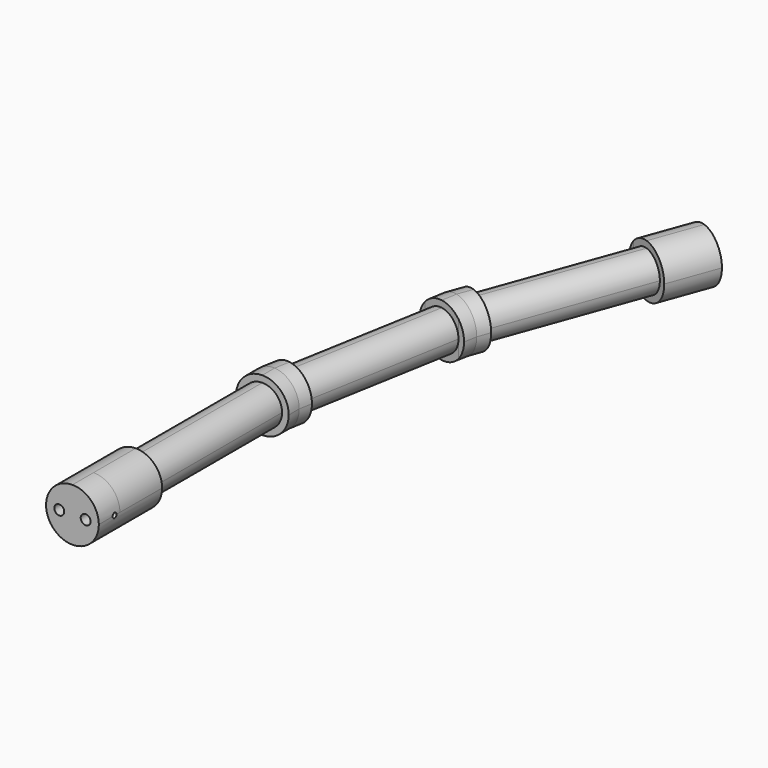
from build123d import *

# Parameters (mm, degrees)
F1_DEPTH  = 25.4
F2_DEPTH  = 19.05
F3_R      = 19.04999
F4_R      = 25.39999
F5_R      = 25.39999
F6_DEPTH  = 25.4
F8_R      = 4.7625
F9_DEPTH  = 25.4
F11_DEPTH = 25.4


# Not quite as in the source:
# - a fillet or chamfer is up to 0.001 mm smaller than in the source, because OpenCascade refuses the exact size
# - a feature names something its author has since deleted; it is built from what else it names


with BuildPart() as f1:
    # F0 (on Top) → F1 (new body, symmetric)
    with BuildSketch(Plane.XY):
        Polygon((12.8819166735, 369.5075380505), (7.0181782831, 353.3970492294), (56.2746459892, 340.1988184856), (60.6183018094, 352.1329147696), (54.6512536674, 354.3047426797), (18.8489648155, 367.3357101404), align=None)
        Polygon((4.0410802798, 336.5130874478), (10.2946095114, 335.4104215196), (47.8157849012, 328.7944259505), (54.0693141328, 327.6917600223), (56.2746459892, 340.1988184856), (7.0181782831, 353.3970492294), align=None)
    extrude(amount=F1_DEPTH, both=True)



with BuildPart() as f1b:
    # F0 (on Top) → F1, piece 2 (new body, symmetric)
    with BuildSketch(Plane.XY):
        Polygon((-22.4229019967, 186.4283858887), (-25.4, 169.5444241071), (25.4, 165.1), (27.6053318564, 177.6070584633), (21.3518026247, 178.7097243914), (-16.169372765, 185.3257199606), align=None)
        Polygon((-25.4, 152.4), (-19.05, 152.4), (19.05, 152.4), (25.4, 152.4), (25.4, 165.1), (-25.4, 169.5444241071), align=None)
    extrude(amount=F1_DEPTH, both=True)


with BuildPart() as f1c:
    # F0 (on Top) → F1, piece 3 (new body, symmetric)
    with BuildSketch(Plane.XY):
        Polygon((19.05, 0), (0, 0), (-19.05, 0), (-25.4, 0), (-25.4, -50.8), (25.4, -50.8), (25.4, 0), align=None)
    extrude(amount=F1_DEPTH, both=True)


with BuildPart() as f1d:
    # F0 (on Top) → F1, piece 4 (new body, symmetric)
    with BuildSketch(Plane.XY):
        Polygon((65.0057865163, 512.7166934583), (70.9728346583, 510.5448655482), (106.7751235103, 497.5138980874), (112.7421716522, 495.3420701773), (130.1167949332, 543.0784553132), (82.3804097973, 560.4530785942), align=None)
    extrude(amount=F1_DEPTH, both=True)


with BuildPart() as f1_1:
    add(f1.part)

    add(f1b.part)  # F2 merges F1b

    add(f1c.part)  # F2 merges F1c

    add(f1d.part)  # F2 merges F1d
    # F0 (on Top) → F2 (join, symmetric)
    with BuildSketch(Plane.XY):
        Polygon((70.9728346583, 510.5448655482), (18.8489648155, 367.3357101404), (54.6512536674, 354.3047426797), (106.7751235103, 497.5138980874), align=None)
        Polygon((10.2946095114, 335.4104215196), (-16.169372765, 185.3257199606), (21.3518026247, 178.7097243914), (47.8157849012, 328.7944259505), align=None)
        Polygon((-19.05, 0), (0, 0), (19.05, 0), (19.05, 152.4), (-19.05, 152.4), align=None)
    extrude(amount=F2_DEPTH, both=True)

    # F3 (radius 19.05 in the source; OpenCascade refuses exactly that, so slightly less here)
    f3_edges = [f1_1.edges().sort_by_distance(p)[0] for p in [
        (80.713189, 425.90932, 19.05),
        (44.9109, 438.940288, 19.05),
        (34.583794, 253.752075, 19.05),
        (-2.937382, 260.368071, 19.05),
        (19.05, 76.2, 19.05),
        (-19.05, 76.2, 19.05),
        (19.05, 76.2, -19.05),
        (-19.05, 76.2, -19.05),
        (34.583794, 253.752075, -19.05),
        (-2.937382, 260.368071, -19.05),
        (80.713189, 425.90932, -19.05),
        (44.9109, 438.940288, -19.05),
    ]]
    fillet(f3_edges, radius=F3_R)

    # F4 (radius 25.4 in the source; OpenCascade refuses exactly that, so slightly less here)
    f4_edges = [f1_1.edges().sort_by_distance(p)[0] for p in [
        (26.502666, 171.353529, 25.4),
        (-23.911451, 177.986405, 25.4),
        (-25.4, 160.972212, 25.4),
        (25.4, 158.75, 25.4),
        (26.502666, 171.353529, -25.4),
        (25.4, 158.75, -25.4),
        (-25.4, 160.972212, -25.4),
        (-23.911451, 177.986405, -25.4),
        (5.529629, 344.955068, -25.4),
        (9.950047, 361.452294, -25.4),
        (55.17198, 333.945289, -25.4),
        (58.446474, 346.165867, -25.4),
        (58.446474, 346.165867, 25.4),
        (9.950047, 361.452294, 25.4),
        (5.529629, 344.955068, 25.4),
        (55.17198, 333.945289, 25.4),
        (121.429483, 519.210263, 25.4),
        (121.429483, 519.210263, -25.4),
        (73.693098, 536.584886, 25.4),
        (73.693098, 536.584886, -25.4),
    ]]
    fillet(f4_edges, radius=F4_R)

    # F5 (radius 25.4 in the source; OpenCascade refuses exactly that, so slightly less here)
    f5_edges = [f1_1.edges().sort_by_distance(p)[0] for p in [
        (-25.4, -25.4, -25.4),
        (25.4, -25.4, -25.4),
        (-25.4, -25.4, 25.4),
        (25.4, -25.4, 25.4),
    ]]
    fillet(f5_edges, radius=F5_R)

    # F6 (add): a face of the model
    f6_faces = [f1_1.faces().sort_by_distance(p)[0] for p in [
        (0, -50.8, 0),
    ]]
    extrude(f6_faces, amount=F6_DEPTH)

    # F8 (on face) → F9 (cut)
    with BuildSketch(Plane.XZ.offset(76.2)):
        with Locations((-12.7, 0)):
            Circle(F8_R)
        with BuildLine():
            ThreePointArc((17.4625, 0), (12.7, 4.7625), (7.9375, 0))
            ThreePointArc((7.9375, 0), (12.7, -4.7625), (17.4625, 0))
        make_face()
    extrude(amount=-F9_DEPTH, mode=Mode.SUBTRACT)

    # F10 (on Right) → F11 (cut, symmetric)
    with BuildSketch(Plane.YZ):
        with BuildLine():
            ThreePointArc((-59.53125, 0), (-57.15, -2.38125), (-54.76875, 0))
            ThreePointArc((-54.76875, 0), (-57.15, 2.38125), (-59.53125, 0))
        make_face()
    extrude(amount=F11_DEPTH, both=True, mode=Mode.SUBTRACT)


solid = f1_1.part
